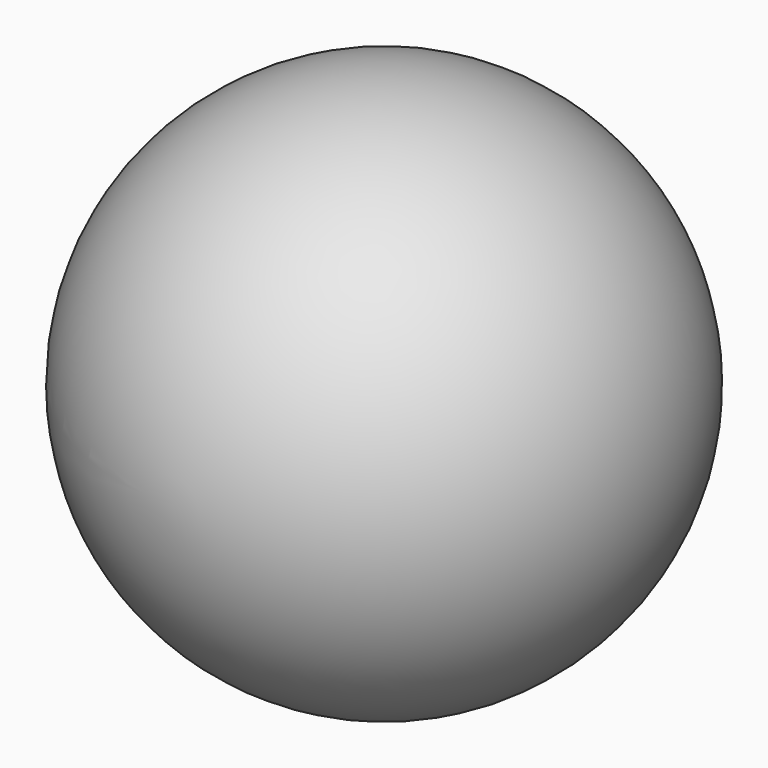
from build123d import *

# Parameters (mm, degrees)
F0_R = 4.9490069848


# Not quite as in the source:
# - the program builds the solid bodies; features that only make, move or delete a surface that nothing else refers to are left out


with BuildPart() as f1:
    # F0 (on Top) → F1 (revolve)
    with BuildSketch(Plane.XY):
        with BuildLine():
            Line((0, -32.6587968732), (0, 32.6587968732))
            ThreePointArc((0, 32.6587968732), (-32.6587968732, 0), (0, -32.6587968732))
        make_face()
        with BuildLine():
            Line((0, 32.6587968732), (0, 54.7258222024))
            ThreePointArc((0, 54.7258222024), (-54.7258222024, 0), (0, -54.7258222024))
            Line((0, -54.7258222024), (0, -32.6587968732))
            ThreePointArc((0, -32.6587968732), (-32.6587968732, 0), (0, 32.6587968732))
        make_face()
        with Locations((-43.5705259442, -0.5094259977)):
            Circle(F0_R, mode=Mode.SUBTRACT)
    revolve(axis=Axis((0, 0, 0), (0, -1, 0)))


solid = f1.part
